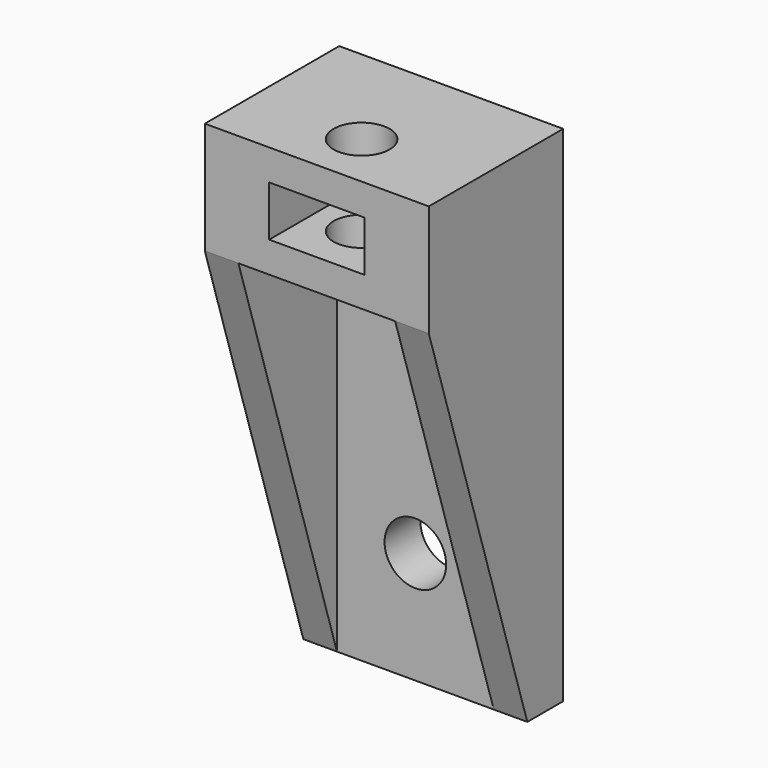
from build123d import *

# Parameters (mm, degrees)
F0_W     = 20
F0_H     = 40
F0_R     = 2.75
F1_DEPTH = 4
F2_W     = 20
F2_H     = 10
F3_DEPTH = 15
F4_W     = 8.5
F4_H     = 4.5
F5_DEPTH = 30
F6_R     = 2.5
F7_DEPTH = 20
F9_DEPTH = 3


# Not quite as in the source:
# - a pattern or mirror of a feature is missing from the dataset's text; its kind, count and spacing are read off the source's solid


with BuildPart() as f1:
    # F0 (on Front) → F1 (new body)
    with BuildSketch(Plane.XZ):
        Rectangle(F0_W, F0_H)
        with Locations((0, -10)):
            Circle(F0_R, mode=Mode.SUBTRACT)
        with Locations((0, 10)):
            Circle(F0_R, mode=Mode.SUBTRACT)
    extrude(amount=F1_DEPTH)

    # F2 (on face) → F3 (join)
    with BuildSketch(Plane(origin=(0, 0, 0), x_dir=(-1, 0, 0), z_dir=(0, 1, 0))):
        with Locations((0, 20)):
            Rectangle(F2_W, F2_H)
    extrude(amount=-F3_DEPTH)

    # F4 (on face) → F5 (cut)
    with BuildSketch(Plane.XZ.offset(15)):
        with Locations((0, 20)):
            Rectangle(F4_W, F4_H)
    extrude(amount=-F5_DEPTH, mode=Mode.SUBTRACT)

    # F6 (on face) → F7 (cut)
    with BuildSketch(Plane.XY.offset(25)):
        with Locations((0, -10)):
            Circle(F6_R)
    extrude(amount=-F7_DEPTH, mode=Mode.SUBTRACT)

    # F8 (on face) → F9 (join)
    with BuildSketch(Plane(origin=(-10, 0, 0), x_dir=(0, -1, 0), z_dir=(-1, 0, 0))):
        Polygon((4, -20), (15, 15), (4, 15), align=None)
    f9 = extrude(amount=-F9_DEPTH)

    # F9_copies: F9 across plane
    add(f9.mirror(Plane(origin=(0, 0, 0), x_dir=(0, 0, 1), z_dir=(1, 0, 0))))


solid = f1.part
